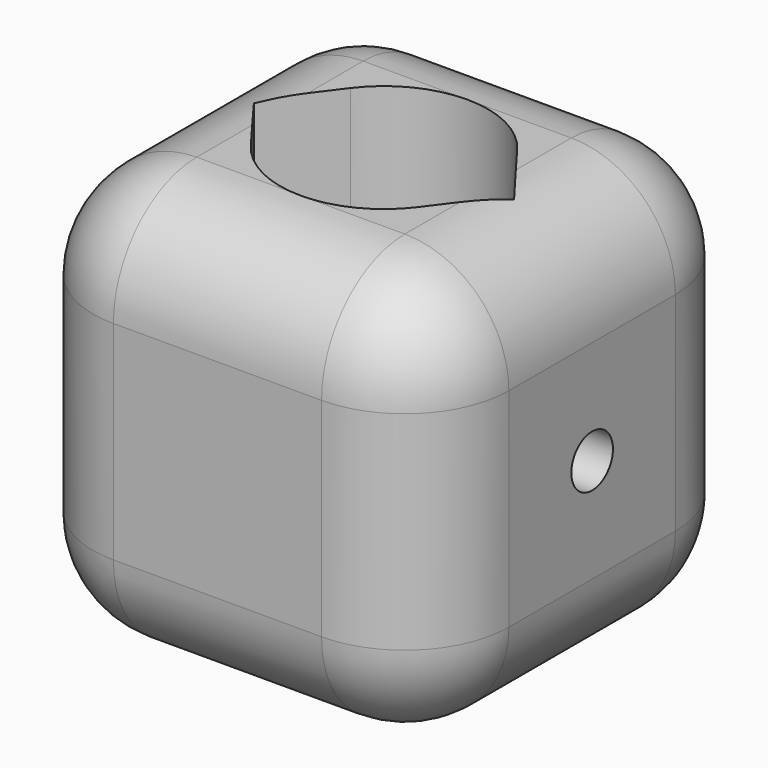
from build123d import *

# Parameters (mm, degrees)
F0_W         = 12.7
F0_H         = 12.7
F1_DEPTH     = 12.7
F2_T1_DEPTH  = 6.35
F2_T3_DEPTH  = 6.35
F2_T5_DEPTH  = 6.35
F2_S9_W      = 3.175
F2_S9_H      = 3.175
F2_T10_DEPTH = 3.175
F2_S15_W     = 3.175
F2_S15_H     = 3.175
F2_T16_DEPTH = 3.175
F2_S21_W     = 3.175
F2_S21_H     = 3.175
F2_T22_DEPTH = 3.175
F2_S27_W     = 3.175
F2_S27_H     = 3.175
F2_T28_DEPTH = 3.175
F2_S33_W     = 3.175
F2_S33_H     = 3.175
F2_T34_DEPTH = 3.175
F2_S39_W     = 3.175
F2_S39_H     = 3.175
F2_T40_DEPTH = 3.175
F2_S45_W     = 3.175
F2_S45_H     = 3.175
F2_T46_DEPTH = 3.175
F2_S51_W     = 3.175
F2_S51_H     = 3.175
F2_T52_DEPTH = 3.175
F3_R         = 0.79375
F4_DEPTH     = 6.2992


# Not quite as in the source:
# - a fillet or chamfer that OpenCascade refuses, or shapes differently, is made with other operations: its cross-section is extruded or revolved along the edge and cut away or added


with BuildPart() as f1:
    # F0 (on Top) → F1 (new body)
    with BuildSketch(Plane.XY):
        Rectangle(F0_W, F0_H)
        with BuildLine():
            ThreePointArc((-2.54, 1.905), (0, 3.175), (2.54, 1.905))
            Line((2.54, 1.905), (3.96875, 0))
            Line((3.96875, 0), (2.54, -1.905))
            ThreePointArc((2.54, -1.905), (0, -3.175), (-2.54, -1.905))
            Line((-2.54, -1.905), (-3.96875, 0))
            Line((-3.96875, 0), (-2.54, 1.905))
        make_face(mode=Mode.SUBTRACT)
    extrude(amount=F1_DEPTH)

    # F2: fillet of radius 3.175 on 12 edges, made by hand

    # F2_s2 → F2_t1 (cut)
    with BuildSketch(Plane.XY.offset(3.175)):
        with BuildLine():
            ThreePointArc((6.35, -3.175), (5.4200640303, -5.4200640303), (3.175, -6.35))
            Line((3.175, -6.35), (6.35, -6.35))
            Line((6.35, -6.35), (6.35, -3.175))
        make_face()
        with BuildLine():
            ThreePointArc((6.35, 3.175), (5.4200640303, 5.4200640303), (3.175, 6.35))
            Line((3.175, 6.35), (6.35, 6.35))
            Line((6.35, 6.35), (6.35, 3.175))
        make_face()
        with BuildLine():
            ThreePointArc((-3.175, 6.35), (-5.4200640303, 5.4200640303), (-6.35, 3.175))
            Line((-6.35, 3.175), (-6.35, 6.35))
            Line((-6.35, 6.35), (-3.175, 6.35))
        make_face()
        with BuildLine():
            ThreePointArc((-6.35, -3.175), (-5.4200640303, -5.4200640303), (-3.175, -6.35))
            Line((-3.175, -6.35), (-6.35, -6.35))
            Line((-6.35, -6.35), (-6.35, -3.175))
        make_face()
    extrude(amount=F2_T1_DEPTH, mode=Mode.SUBTRACT)

    # F2_s4 → F2_t3 (cut)
    with BuildSketch(Plane.YZ.offset(-3.175)):
        with BuildLine():
            ThreePointArc((-6.35, 9.525), (-5.4200640303, 11.7700640303), (-3.175, 12.7))
            Line((-3.175, 12.7), (-6.35, 12.7))
            Line((-6.35, 12.7), (-6.35, 9.525))
        make_face()
        with BuildLine():
            ThreePointArc((-6.35, 3.175), (-5.4200640303, 0.9299359697), (-3.175, 0))
            Line((-3.175, 0), (-6.35, 0))
            Line((-6.35, 0), (-6.35, 3.175))
        make_face()
        with BuildLine():
            ThreePointArc((6.35, 3.175), (5.4200640303, 0.9299359697), (3.175, 0))
            Line((3.175, 0), (6.35, 0))
            Line((6.35, 0), (6.35, 3.175))
        make_face()
        with BuildLine():
            ThreePointArc((6.35, 9.525), (5.4200640303, 11.7700640303), (3.175, 12.7))
            Line((3.175, 12.7), (6.35, 12.7))
            Line((6.35, 12.7), (6.35, 9.525))
        make_face()
    extrude(amount=F2_T3_DEPTH, mode=Mode.SUBTRACT)

    # F2_s6 → F2_t5 (cut)
    with BuildSketch(Plane.XZ.offset(-3.175)):
        with BuildLine():
            ThreePointArc((6.35, 9.525), (5.4200640303, 11.7700640303), (3.175, 12.7))
            Line((3.175, 12.7), (6.35, 12.7))
            Line((6.35, 12.7), (6.35, 9.525))
        make_face()
        with BuildLine():
            ThreePointArc((6.35, 3.175), (5.4200640303, 0.9299359697), (3.175, 0))
            Line((3.175, 0), (6.35, 0))
            Line((6.35, 0), (6.35, 3.175))
        make_face()
        with BuildLine():
            ThreePointArc((-6.35, 3.175), (-5.4200640303, 0.9299359697), (-3.175, 0))
            Line((-3.175, 0), (-6.35, 0))
            Line((-6.35, 0), (-6.35, 3.175))
        make_face()
        with BuildLine():
            ThreePointArc((-6.35, 9.525), (-5.4200640303, 11.7700640303), (-3.175, 12.7))
            Line((-3.175, 12.7), (-6.35, 12.7))
            Line((-6.35, 12.7), (-6.35, 9.525))
        make_face()
    extrude(amount=F2_T5_DEPTH, mode=Mode.SUBTRACT)


with BuildPart() as f2_tool8:
    # F2_s9 → F2_t10 (new body)
    with BuildSketch(Plane.YZ.offset(3.175)):
        with Locations((-4.7625, 1.5875)):
            Rectangle(F2_S9_W, F2_S9_H)
    extrude(amount=F2_T10_DEPTH)

    # F2_s11 → F2_t12 (revolve, cut)
    with BuildSketch(Plane(origin=(3.175, -3.175, 3.175), x_dir=(0, 0.7071067812, 0.7071067812), z_dir=(0, 0.7071067812, -0.7071067812))):
        with BuildLine():
            ThreePointArc((0, -3.175), (3.175, 0), (0, 3.175))
            Line((0, 3.175), (0, -3.175))
        make_face()
    revolve(axis=Axis((3.175, -3.175, 3.175), (1, 0, 0)), mode=Mode.SUBTRACT)


with BuildPart() as f1_1:
    add(f1.part)

    # F2_t7: cut F2_tool8
    add(f2_tool8.part, mode=Mode.SUBTRACT)


with BuildPart() as f2_tool14:
    # F2_s15 → F2_t16 (new body)
    with BuildSketch(Plane.YZ.offset(3.175)):
        with Locations((-4.7625, 11.1125)):
            Rectangle(F2_S15_W, F2_S15_H)
    extrude(amount=F2_T16_DEPTH)

    # F2_s17 → F2_t18 (revolve, cut)
    with BuildSketch(Plane(origin=(3.175, -3.175, 9.525), x_dir=(0, 0.7071067812, -0.7071067812), z_dir=(0, -0.7071067812, -0.7071067812))):
        with BuildLine():
            ThreePointArc((0, -3.175), (3.175, 0), (0, 3.175))
            Line((0, 3.175), (0, -3.175))
        make_face()
    revolve(axis=Axis((3.175, -3.175, 9.525), (1, 0, 0)), mode=Mode.SUBTRACT)


with BuildPart() as f1_2:
    add(f1_1.part)

    # F2_t13: cut F2_tool14
    add(f2_tool14.part, mode=Mode.SUBTRACT)


with BuildPart() as f2_tool20:
    # F2_s21 → F2_t22 (new body)
    with BuildSketch(Plane.XY.offset(9.525)):
        with Locations((-4.7625, -4.7625)):
            Rectangle(F2_S21_W, F2_S21_H)
    extrude(amount=F2_T22_DEPTH)

    # F2_s23 → F2_t24 (revolve, cut)
    with BuildSketch(Plane(origin=(-3.175, -3.175, 9.525), x_dir=(0.7071067812, 0.7071067812, 0), z_dir=(0.7071067812, -0.7071067812, 0))):
        with BuildLine():
            ThreePointArc((0, -3.175), (3.175, 0), (0, 3.175))
            Line((0, 3.175), (0, -3.175))
        make_face()
    revolve(axis=Axis((-3.175, -3.175, 9.525), (0, 0, 1)), mode=Mode.SUBTRACT)


with BuildPart() as f1_3:
    add(f1_2.part)

    # F2_t19: cut F2_tool20
    add(f2_tool20.part, mode=Mode.SUBTRACT)


with BuildPart() as f2_tool26:
    # F2_s27 → F2_t28 (new body)
    with BuildSketch(Plane.YZ.offset(3.175)):
        with Locations((4.7625, 11.1125)):
            Rectangle(F2_S27_W, F2_S27_H)
    extrude(amount=F2_T28_DEPTH)

    # F2_s29 → F2_t30 (revolve, cut)
    with BuildSketch(Plane(origin=(3.175, 3.175, 9.525), x_dir=(0, -0.7071067812, -0.7071067812), z_dir=(0, -0.7071067812, 0.7071067812))):
        with BuildLine():
            ThreePointArc((0, -3.175), (3.175, 0), (0, 3.175))
            Line((0, 3.175), (0, -3.175))
        make_face()
    revolve(axis=Axis((3.175, 3.175, 9.525), (1, 0, 0)), mode=Mode.SUBTRACT)


with BuildPart() as f1_4:
    add(f1_3.part)

    # F2_t25: cut F2_tool26
    add(f2_tool26.part, mode=Mode.SUBTRACT)


with BuildPart() as f2_tool32:
    # F2_s33 → F2_t34 (new body)
    with BuildSketch(Plane.YZ.offset(3.175)):
        with Locations((4.7625, 1.5875)):
            Rectangle(F2_S33_W, F2_S33_H)
    extrude(amount=F2_T34_DEPTH)

    # F2_s35 → F2_t36 (revolve, cut)
    with BuildSketch(Plane(origin=(3.175, 3.175, 3.175), x_dir=(0, -0.7071067812, 0.7071067812), z_dir=(0, 0.7071067812, 0.7071067812))):
        with BuildLine():
            ThreePointArc((0, -3.175), (3.175, 0), (0, 3.175))
            Line((0, 3.175), (0, -3.175))
        make_face()
    revolve(axis=Axis((3.175, 3.175, 3.175), (1, 0, 0)), mode=Mode.SUBTRACT)


with BuildPart() as f1_5:
    add(f1_4.part)

    # F2_t31: cut F2_tool32
    add(f2_tool32.part, mode=Mode.SUBTRACT)


with BuildPart() as f2_tool38:
    # F2_s39 → F2_t40 (new body)
    with BuildSketch(Plane.YZ.offset(-3.175)):
        with Locations((-4.7625, 1.5875)):
            Rectangle(F2_S39_W, F2_S39_H)
    extrude(amount=-F2_T40_DEPTH)

    # F2_s41 → F2_t42 (revolve, cut)
    with BuildSketch(Plane(origin=(-3.175, -3.175, 3.175), x_dir=(0, 0.7071067812, 0.7071067812), z_dir=(0, -0.7071067812, 0.7071067812))):
        with BuildLine():
            ThreePointArc((0, -3.175), (3.175, 0), (0, 3.175))
            Line((0, 3.175), (0, -3.175))
        make_face()
    revolve(axis=Axis((-3.175, -3.175, 3.175), (-1, 0, 0)), mode=Mode.SUBTRACT)


with BuildPart() as f1_6:
    add(f1_5.part)

    # F2_t37: cut F2_tool38
    add(f2_tool38.part, mode=Mode.SUBTRACT)


with BuildPart() as f2_tool44:
    # F2_s45 → F2_t46 (new body)
    with BuildSketch(Plane.XZ.offset(-3.175)):
        with Locations((-4.7625, 1.5875)):
            Rectangle(F2_S45_W, F2_S45_H)
    extrude(amount=-F2_T46_DEPTH)

    # F2_s47 → F2_t48 (revolve, cut)
    with BuildSketch(Plane(origin=(-3.175, 3.175, 3.175), x_dir=(0.7071067812, 0, 0.7071067812), z_dir=(-0.7071067812, 0, 0.7071067812))):
        with BuildLine():
            ThreePointArc((0, -3.175), (3.175, 0), (0, 3.175))
            Line((0, 3.175), (0, -3.175))
        make_face()
    revolve(axis=Axis((-3.175, 3.175, 3.175), (0, 1, 0)), mode=Mode.SUBTRACT)


with BuildPart() as f1_7:
    add(f1_6.part)

    # F2_t43: cut F2_tool44
    add(f2_tool44.part, mode=Mode.SUBTRACT)


with BuildPart() as f2_tool50:
    # F2_s51 → F2_t52 (new body)
    with BuildSketch(Plane.XZ.offset(-3.175)):
        with Locations((-4.7625, 11.1125)):
            Rectangle(F2_S51_W, F2_S51_H)
    extrude(amount=-F2_T52_DEPTH)

    # F2_s53 → F2_t54 (revolve, cut)
    with BuildSketch(Plane(origin=(-3.175, 3.175, 9.525), x_dir=(0.7071067812, 0, -0.7071067812), z_dir=(0.7071067812, 0, 0.7071067812))):
        with BuildLine():
            ThreePointArc((0, -3.175), (3.175, 0), (0, 3.175))
            Line((0, 3.175), (0, -3.175))
        make_face()
    revolve(axis=Axis((-3.175, 3.175, 9.525), (0, 1, 0)), mode=Mode.SUBTRACT)


with BuildPart() as f1_8:
    add(f1_7.part)

    # F2_t49: cut F2_tool50
    add(f2_tool50.part, mode=Mode.SUBTRACT)

    # F3 (on face) → F4 (cut)
    with BuildSketch(Plane.YZ.offset(6.35)):
        with Locations((0, 6.35)):
            Circle(F3_R)
    extrude(amount=-F4_DEPTH, mode=Mode.SUBTRACT)


solid = f1_8.part
